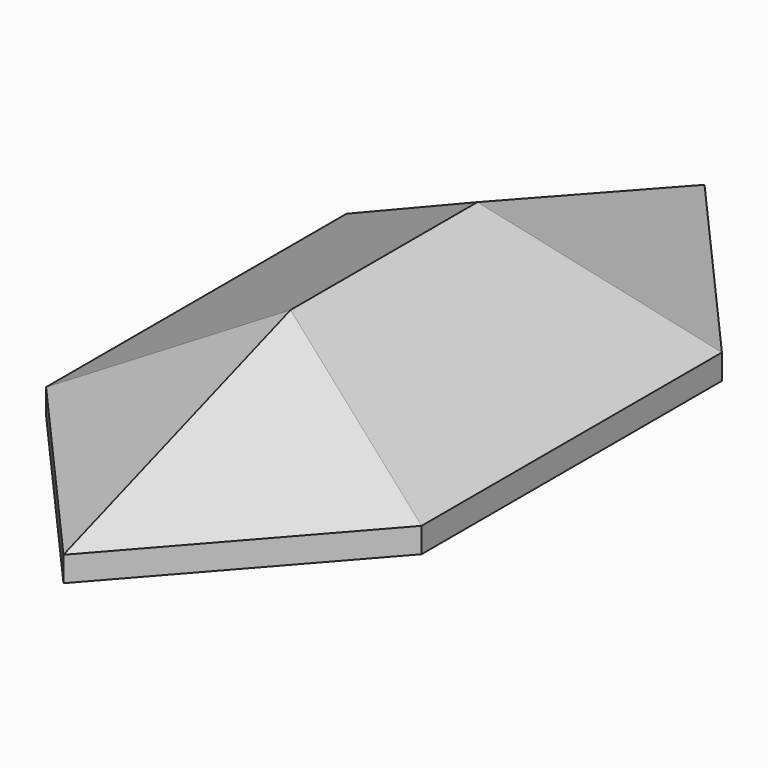
from build123d import *

# Parameters (mm, degrees)
F0_W     = 7.62
F0_H     = 7.62
F1_DEPTH = 2.54
F2_SIZE2 = 3.80999
F2_SIZE  = 2.03199
F3_T     = -0.762


# Not quite as in the source:
# - a fillet or chamfer is up to 0.001 mm smaller than in the source, because OpenCascade refuses the exact size


with BuildPart() as f1:
    # F0 (on Top) → F1 (new body)
    with BuildSketch(Plane.XY):
        Rectangle(F0_W, F0_H)
        Polygon((-3.81, 3.81), (3.81, 3.81), (0, 8.1314574927), align=None)
        Polygon((0, -8.1314574927), (3.81, -3.81), (-3.81, -3.81), align=None)
    extrude(amount=F1_DEPTH)

    # F2 (size 2.032 and 3.81 in the source; OpenCascade refuses exactly that, so slightly less here)
    f2_edges = [f1.edges().sort_by_distance(p)[0] for p in [
        (3.81, 0, 2.54),
        (1.905, 5.970729, 2.54),
        (-1.905, -5.970729, 2.54),
        (-3.81, 0, 2.54),
        (-1.905, 5.970729, 2.54),
        (1.905, -5.970729, 2.54),
    ]]
    chamfer(f2_edges, length=F2_SIZE, length2=F2_SIZE2)

    # F3
    f3_openings = [f1.faces().sort_by_distance(p)[0] for p in [
        (0, 0, 0),
    ]]
    offset(amount=F3_T, openings=f3_openings)


solid = f1.part
